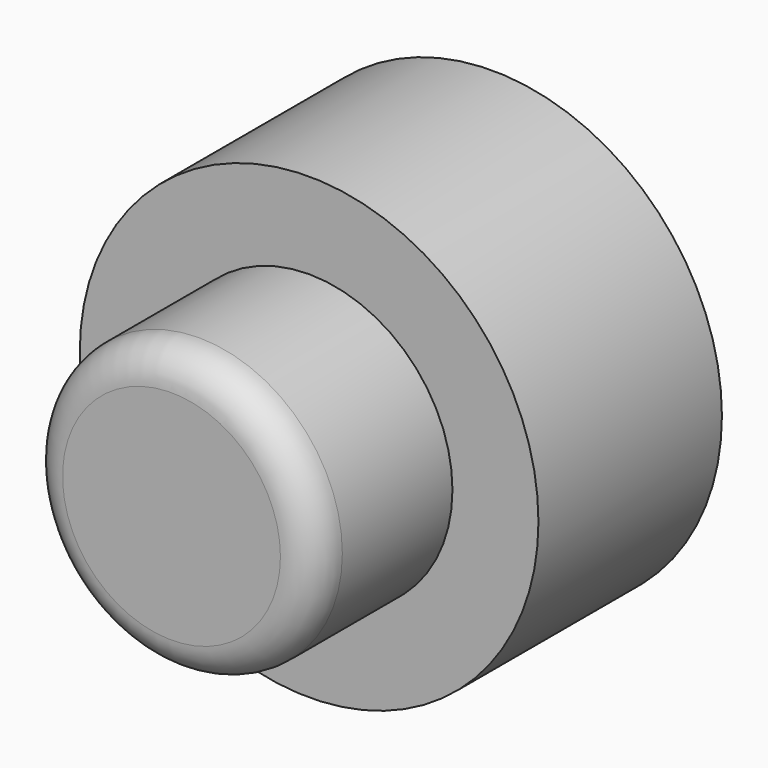
from build123d import *

# Parameters (mm, degrees)
F0_R     = 1.65
F1_DEPTH = 7
F0_R_2   = 2.5
F2_DEPTH = 7
F0_R_3   = 4
F3_DEPTH = 4
F4_R     = 0.6


with BuildPart() as f1:
    # F0 (on Front) → F1 (new body)
    with BuildSketch(Plane.XZ):
        Circle(F0_R)
    extrude(amount=F1_DEPTH)

    # F0 (on Front) → F2 (join)
    with BuildSketch(Plane.XZ):
        Circle(F0_R_2)
        Circle(F0_R, mode=Mode.SUBTRACT)
    extrude(amount=F2_DEPTH)

    # F0 (on Front) → F3 (join)
    with BuildSketch(Plane.XZ):
        Circle(F0_R_3)
        Circle(F0_R_2, mode=Mode.SUBTRACT)
    extrude(amount=F3_DEPTH)

    # F4
    f4_edges = [f1.edges().sort_by_distance(p)[0] for p in [
        (-2.5, -7, 0),
    ]]
    fillet(f4_edges, radius=F4_R)


solid = f1.part
